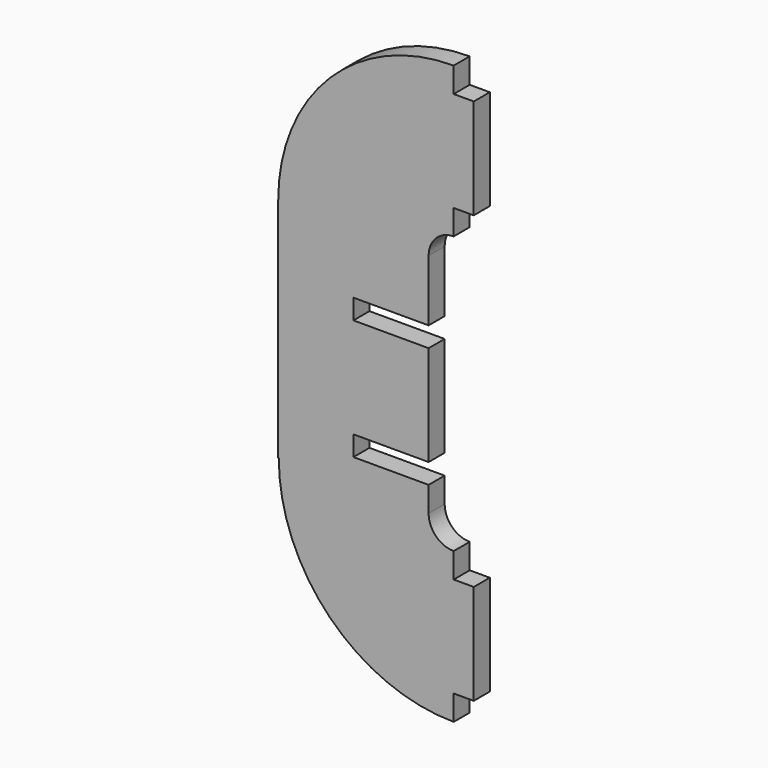
from build123d import *

# Parameters (mm, degrees)
F0_W     = 8
F0_H     = 40
F1_DEPTH = 8


# Not quite as in the source:
# - ends of sketch curves that miss each other by under 0.0002 mm in the source are joined


with BuildPart() as f1:
    # F0 (on Front) → F1 (new body)
    with BuildSketch(Plane.XZ):
        with Locations((44, 85.25)):
            Rectangle(F0_W, F0_H)
        with Locations((44, -85.25)):
            Rectangle(F0_W, F0_H)
        with BuildLine():
            Line((30, -45.25), (-29.7788833363, -45.25))
            ThreePointArc((-29.7788833363, -45.25), (-9.3545962046, -94.6694618691), (40, -115.25))
            Line((40, -115.25), (40, -105.25))
            Line((40, -105.25), (40, -65.25))
            Line((40, -65.25), (40, -55.25))
            ThreePointArc((40, -55.25), (32.9289321881, -52.3210678119), (30, -45.25))
        make_face()
        with BuildLine():
            ThreePointArc((40, 115.25), (-9.4974751888, 94.7474741773), (-30, 45.2499985695))
            Line((-30, 45.2499985695), (30, 45.25))
            ThreePointArc((30, 45.25), (32.9289321881, 52.3210678119), (40, 55.25))
            Line((40, 55.25), (40, 65.25))
            Line((40, 65.25), (40, 105.25))
            Line((40, 105.25), (40, 115.25))
        make_face()
        Polygon((-30, 45.25), (-30, -45.25), (-29.7788833363, -45.25), (30, -45.25), (30, -35.25), (0, -35.25), (0, -27.25), (30, -27.25), (30, 12.75), (0, 12.75), (0, 20.75), (30, 20.75), (30, 45.25), align=None)
    extrude(amount=F1_DEPTH)


solid = f1.part
